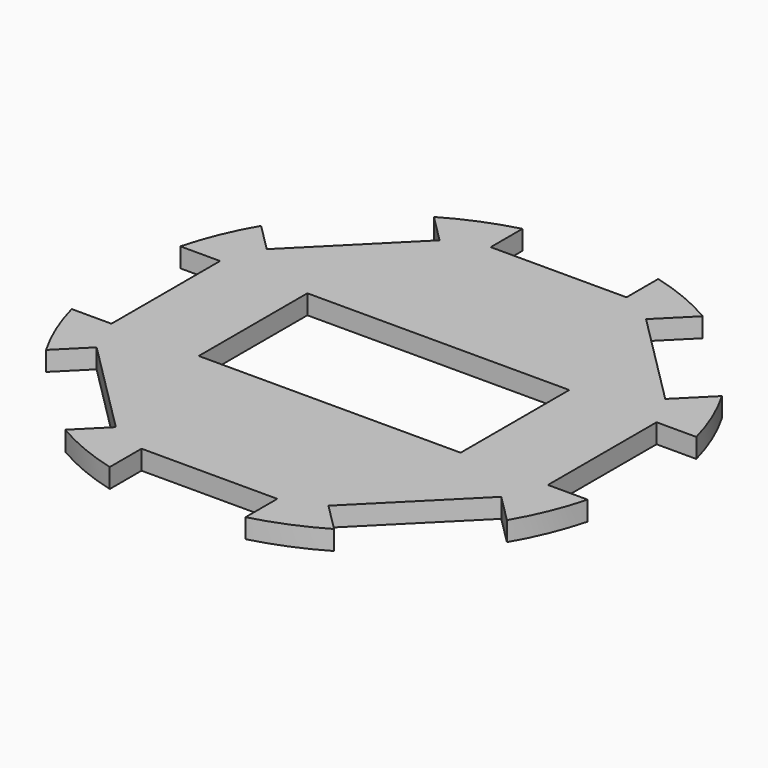
from build123d import *

# Parameters (mm, degrees)
F0_W     = 54
F0_H     = 28
F1_DEPTH = 4


# Not quite as in the source:
# - a feature of the source that left no trace in its solid (it failed there, or was rolled back) is left out


with BuildPart() as f1:
    # F0 (on Top) → F1 (new body)
    with BuildSketch(Plane.XY):
        with BuildLine():
            Line((14, -45), (14, -53.1883445879))
            ThreePointArc((14, -53.1883445879), (21.0475887801, -50.8133742881), (27.7103442016, -47.5093340748))
            Line((27.7103442016, -47.5093340748), (21.9203102168, -41.71930009))
            Line((21.9203102168, -41.71930009), (41.71930009, -21.9203102168))
            Line((41.71930009, -21.9203102168), (47.5093340748, -27.7103442016))
            ThreePointArc((47.5093340748, -27.7103442016), (50.8133742881, -21.0475887801), (53.1883445879, -14))
            Line((53.1883445879, -14), (45, -14))
            Line((45, -14), (45, 14))
            Line((45, 14), (53.1883445879, 14))
            ThreePointArc((53.1883445879, 14), (50.8133742881, 21.0475887801), (47.5093340748, 27.7103442016))
            Line((47.5093340748, 27.7103442016), (41.0177921349, 21.2188022616))
            Line((41.0177921349, 21.2188022616), (21.2188022616, 41.0177921349))
            Line((21.2188022616, 41.0177921349), (27.7103442016, 47.5093340748))
            ThreePointArc((27.7103442016, 47.5093340748), (21.0475887801, 50.8133742881), (14, 53.1883445879))
            Line((14, 53.1883445879), (14, 45))
            Line((14, 45), (-14, 45))
            Line((-14, 45), (-14, 53.1883445879))
            ThreePointArc((-14, 53.1883445879), (-21.0475887801, 50.8133742881), (-27.7103442016, 47.5093340748))
            Line((-27.7103442016, 47.5093340748), (-21.9203102168, 41.71930009))
            Line((-21.9203102168, 41.71930009), (-41.71930009, 21.9203102168))
            Line((-41.71930009, 21.9203102168), (-47.5093340748, 27.7103442016))
            ThreePointArc((-47.5093340748, 27.7103442016), (-50.8133742881, 21.0475887801), (-53.1883445879, 14))
            Line((-53.1883445879, 14), (-45, 14))
            Line((-45, 14), (-45, -14))
            Line((-45, -14), (-53.1883445879, -14))
            ThreePointArc((-53.1883445879, -14), (-50.8133742881, -21.0475887801), (-47.5093340748, -27.7103442016))
            Line((-47.5093340748, -27.7103442016), (-41.71930009, -21.9203102168))
            Line((-41.71930009, -21.9203102168), (-21.9203102168, -41.71930009))
            Line((-21.9203102168, -41.71930009), (-27.7103442016, -47.5093340748))
            ThreePointArc((-27.7103442016, -47.5093340748), (-21.0475887801, -50.8133742881), (-14, -53.1883445879))
            Line((-14, -53.1883445879), (-14, -45))
            Line((-14, -45), (14, -45))
        make_face()
        Rectangle(F0_W, F0_H, mode=Mode.SUBTRACT)
    extrude(amount=F1_DEPTH)


solid = f1.part
